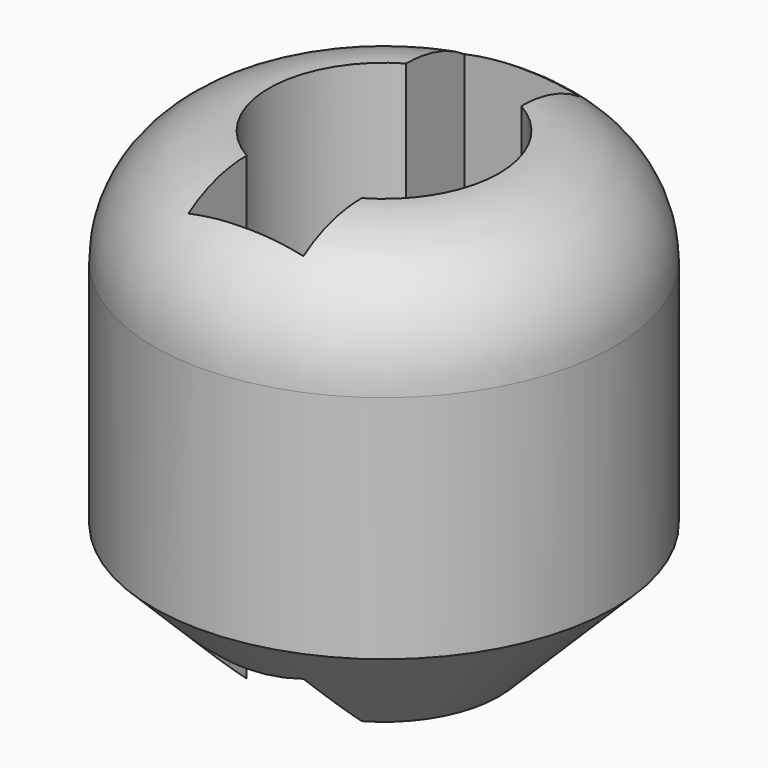
from build123d import *

# Parameters (mm, degrees)
F0_R     = 10
F0_R_2   = 5
F1_DEPTH = 10
F3_DEPTH = 25
F7_D     = 5
F7_DEPTH = 10.0010001


# Not quite as in the source:
# - a fillet or chamfer that OpenCascade refuses, or shapes differently, is made with other operations: its cross-section is extruded or revolved along the edge and cut away or added


with BuildPart() as f1:
    # F0 (on Top) → F1 (new body, symmetric)
    with BuildSketch(Plane.XY):
        Circle(F0_R)
        Circle(F0_R_2, mode=Mode.SUBTRACT)
    extrude(amount=F1_DEPTH, both=True)

    # F2 (on face) → F3 (cut)
    with BuildSketch(Plane.XY.offset(10)):
        with BuildLine():
            Line((2.5, -4.3301270189), (2.5, 4.3301270189))
            ThreePointArc((2.5, 4.3301270189), (0, 5), (-2.5, 4.3301270189))
            Line((-2.5, 4.3301270189), (-2.5, -4.3301270189))
            ThreePointArc((-2.5, -4.3301270189), (0, -5), (2.5, -4.3301270189))
        make_face()
        with BuildLine():
            Line((2.5, 4.3301270189), (2.5, 7.5))
            Line((2.5, 7.5), (-2.5, 7.5))
            Line((-2.5, 7.5), (-2.5, 4.3301270189))
            ThreePointArc((-2.5, 4.3301270189), (0, 5), (2.5, 4.3301270189))
        make_face()
        with BuildLine():
            Line((2.5, -7.5), (2.5, -4.3301270189))
            ThreePointArc((2.5, -4.3301270189), (0, -5), (-2.5, -4.3301270189))
            Line((-2.5, -4.3301270189), (-2.5, -7.5))
            Line((-2.5, -7.5), (2.5, -7.5))
        make_face()
    extrude(amount=-F3_DEPTH, mode=Mode.SUBTRACT)

    # F4: fillet of radius 5 on 1 edges, made by hand

    # F4_s1 → F4_t2 (revolve, cut)
    with BuildSketch(Plane.XZ):
        with BuildLine():
            ThreePointArc((10, 5), (8.5355339059, 8.5355339059), (5, 10))
            Line((5, 10), (10, 10))
            Line((10, 10), (10, 5))
        make_face()
    revolve(axis=Axis((0, 0, 10), (0, 0, 1)), mode=Mode.SUBTRACT)

    # F5: chamfer of 5 on 1 edges, made by hand

    # F5_s1 → F5_t2 (revolve, cut)
    with BuildSketch(Plane.XZ):
        Polygon((10, -5), (5, -10), (10, -10), align=None)
    revolve(axis=Axis((0, 0, -10), (0, 0, 1)), mode=Mode.SUBTRACT)

    # F7 (through all, one way)
    with BuildSketch(Plane.XZ):
        with Locations((0, 0)):
            Circle(F7_D / 2)
    extrude(amount=-F7_DEPTH, mode=Mode.SUBTRACT)


solid = f1.part
